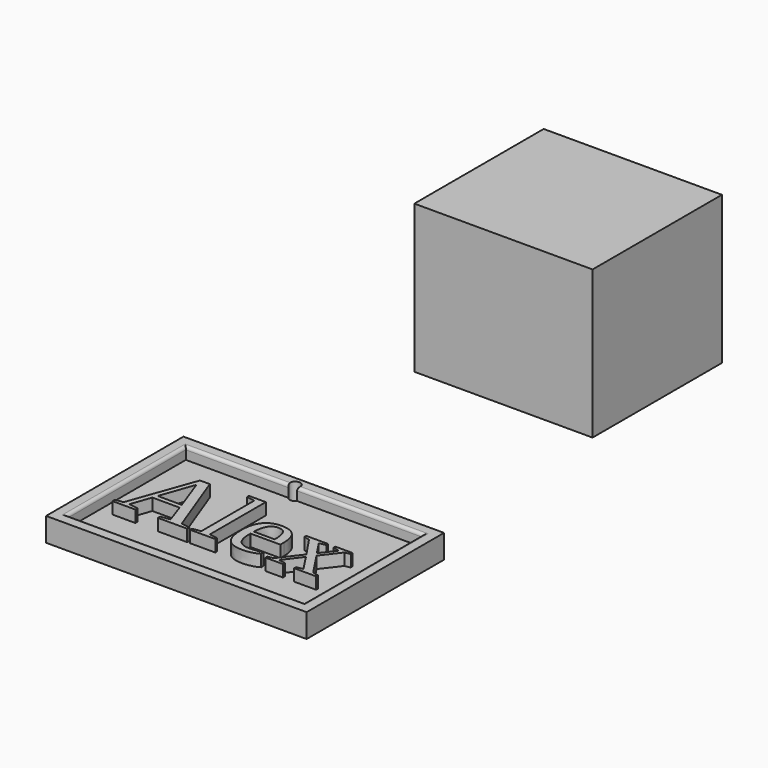
from build123d import *

# Parameters (mm, degrees)
F1_W         = 44
F1_H         = 29
F1_W_2       = 40
F1_H_2       = 25
F2_DEPTH     = 4
F0_W         = 40
F0_H         = 25
F3_DEPTH     = 2
F4_R         = 0.5
F5_TEXT_SIZE = 17.8897397644
F6_DEPTH     = 2
F7_R         = 0.8791958702
F8_DEPTH     = 25
F9_W         = 30.0964079797
F9_H         = 27.3052677512
F10_DEPTH    = 25


# Not quite as in the source:
# - Text() gives the source's letters only with a copy of the font that has no kerning and outlines rounded to 1/6400 em; it was checked with that copy


with BuildPart() as f2:
    # F1 (on face) → F2 (new body)
    with BuildSketch(Plane.XY):
        Rectangle(F1_W, F1_H)
        Rectangle(F1_W_2, F1_H_2, mode=Mode.SUBTRACT)
    extrude(amount=F2_DEPTH)

    # F0 (on Top) → F3 (join)
    with BuildSketch(Plane.XY):
        Rectangle(F0_W, F0_H)
    extrude(amount=F3_DEPTH)

    # F4
    f4_edges = [f2.edges().sort_by_distance(p)[0] for p in [
        (0, 12.5, 4),
        (-20, 0, 4),
        (0, -12.5, 4),
        (20, 0, 4),
    ]]
    fillet(f4_edges, radius=F4_R)

    # F5 (on face) → F6 (join)
    with BuildSketch(Plane.XY.offset(2)):
        with Locations((-17.9671888254, -5.7309769327)):
            Text('Alex', F5_TEXT_SIZE, font='Tinos', text_align=(TextAlign.LEFT, TextAlign.BOTTOM))
    extrude(amount=F6_DEPTH)

    # F7 (on face) → F8 (cut)
    with BuildSketch(Plane.XY.offset(4)):
        with Locations((-1.9445702201, 13)):
            Circle(F7_R)
    extrude(amount=-F8_DEPTH, mode=Mode.SUBTRACT)


with BuildPart() as f10:
    # F9 (on Top) → F10 (new body)
    with BuildSketch(Plane.XY):
        with Locations((0.4558768123, 67.627672106)):
            Rectangle(F9_W, F9_H)
    extrude(amount=F10_DEPTH)


solid = Compound([f2.part, f10.part])
